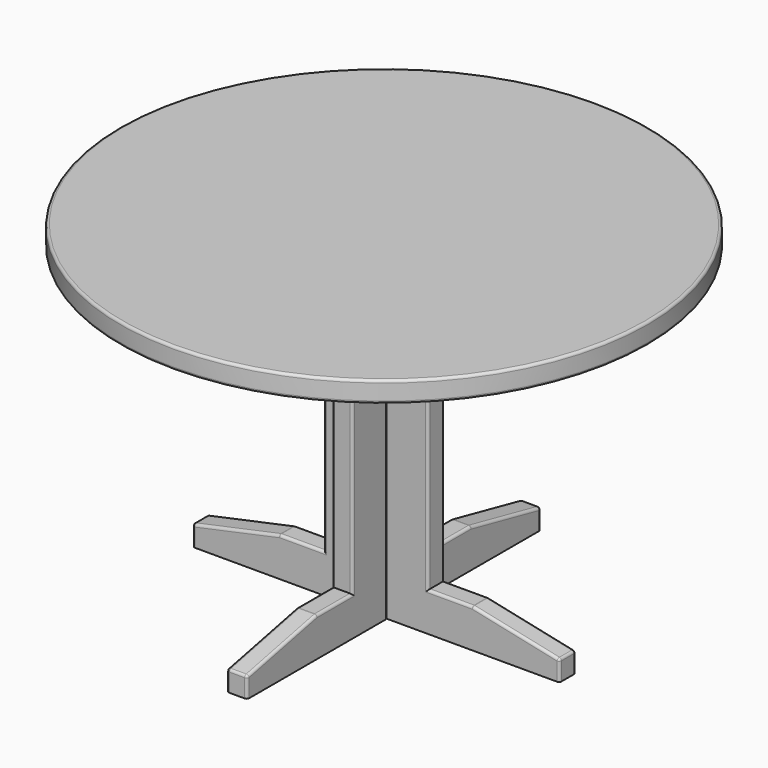
from build123d import *

# Parameters (mm, degrees)
F0_R     = 520.7
F0_W     = 41.275
F0_H     = 256.3125
F0_W_2   = 256.3125
F0_H_2   = 41.275
F0_H_3   = 85
F0_W_3   = 85
F1_DEPTH = 41.275
F2_W     = 82.5
F2_H     = 473.8182766121
F3_DEPTH = 20
F2_H_2   = 474.3196274297
F4_W     = 82.5
F4_H     = 474.3196274297
F5_DEPTH = 20
F4_H_2   = 473.6138966055
F6_R     = 5.08
F6_2_R   = 5.08
F6_3_R   = 5.08
F6_4_R   = 5.08
F6_5_R   = 5.08


# Not quite as in the source:
# - a feature names something its author has since deleted; it is built from what else it names


with BuildPart() as f1:
    # F0 (on Top) → F1 (new body)
    with BuildSketch(Plane.XY):
        Circle(F0_R)
        Polygon((-20.6375, 361.95), (20.6375, 361.95), (20.6375, 105.6375), (20.6375, 20.6375), (105.6375, 20.6375), (361.95, 20.6375), (361.95, -20.6375), (105.6375, -20.6375), (20.6375, -20.6375), (20.6375, -105.6375), (20.6375, -361.95), (-20.6375, -361.95), (-20.6375, -105.6375), (-20.6375, -20.6375), (-105.6375, -20.6375), (-361.95, -20.6375), (-361.95, 20.6375), (-105.6375, 20.6375), (-20.6375, 20.6375), (-20.6375, 105.6375), align=None, mode=Mode.SUBTRACT)
        with Locations((0, 233.79375)):
            Rectangle(F0_W, F0_H)
        with Locations((-233.79375, 0)):
            Rectangle(F0_W_2, F0_H_2)
        with Locations((0, -233.79375)):
            Rectangle(F0_W, F0_H)
        with Locations((233.79375, 0)):
            Rectangle(F0_W_2, F0_H_2)
        Rectangle(F0_W, F0_H_2)
        with Locations((0, 63.1375)):
            Rectangle(F0_W, F0_H_3)
        with Locations((63.1375, 0)):
            Rectangle(F0_W_3, F0_H_2)
        with Locations((0, -63.1375)):
            Rectangle(F0_W, F0_H_3)
        with Locations((-63.1375, 0)):
            Rectangle(F0_W_3, F0_H_2)
    extrude(amount=F1_DEPTH)

    # F6
    f6_edges = [f1.edges().sort_by_distance(p)[0] for p in [
        (-520.7, 0, 41.275),
        (-520.7, 0, 0),
    ]]
    fillet(f6_edges, radius=F6_R)


with BuildPart() as f3:
    # F2 (on Front) → F3 (new body, symmetric)
    with BuildSketch(Plane.XZ):
        Polygon((-361.8104448189, -628.6917154359), (-190.2660957707, -628.7684989539), (-190.2660957707, -551.8782992659), (-361.8104448189, -588.6917154359), align=None)
        Polygon((-190.2660957707, -628.7684989539), (-20.2660957707, -628.8445912188), (-20.2660957707, -551.8782992659), (-102.7660957707, -551.8782992659), (-190.2660957707, -551.8782992659), align=None)
        Polygon((-102.7660957707, -78.0600226537), (-20.2660957707, -78.0600226537), (-20.2660957707, 0), (-190.2660957707, 0), (-190.2660957707, -78.0600226537), align=None)
        Polygon((-362.0399236679, -40), (-190.2660957707, -78.0600226537), (-190.2660957707, 0), (-362.0399236679, 0), align=None)
        with Locations((-61.5160957707, -314.9691609598)):
            Rectangle(F2_W, F2_H)
    extrude(amount=F3_DEPTH, both=True)

    # F6#4
    f6_4_edges = [f3.edges().sort_by_distance(p)[0] for p in [
        (-276.03827, 20, -570.285007),
        (-146.516096, 20, -551.878299),
        (-102.766096, 20, -314.969161),
        (-146.516096, 20, -78.060023),
        (-276.15301, 20, -59.030011),
        (-276.15301, -20, -59.030011),
        (-146.516096, -20, -78.060023),
        (-362.039924, 20, -20),
        (-361.810445, 20, -608.691715),
        (-361.810445, -20, -608.691715),
        (-361.810445, 0, -588.691715),
        (-362.039924, 0, -40),
        (-362.039924, -20, -20),
        (-276.03827, -20, -570.285007),
        (-146.516096, -20, -551.878299),
        (-190.266096, 0, -551.878299),
        (-102.766096, -20, -314.969161),
    ]]
    fillet(f6_4_edges, radius=F6_4_R)


with BuildPart() as f3b:
    # F2 (on Front) → F3, piece 2 (new body, symmetric)
    with BuildSketch(Plane.XZ):
        Polygon((103.0506108094, -552.45), (20.5506108094, -552.45), (20.5506108094, -628.8628608403), (190.5506108094, -628.9389531052), (190.5506108094, -552.45), align=None)
        Polygon((362.153455615, -589.0157628059), (190.5506108094, -552.45), (190.5506108094, -628.9389531052), (362.153455615, -629.0157628059), align=None)
        Polygon((364.0458583832, 0), (190.5506108094, 0), (190.5506108094, -78.1303725703), (364.0458583832, -40), align=None)
        Polygon((190.5506108094, 0), (20.5506108094, 0), (20.5506108094, -78.1303725703), (103.0506108094, -78.1303725703), (190.5506108094, -78.1303725703), align=None)
        with Locations((61.8006108094, -315.2901862851)):
            Rectangle(F2_W, F2_H_2)
    extrude(amount=F3_DEPTH, both=True)

    # F6#2
    f6_2_edges = [f3b.edges().sort_by_distance(p)[0] for p in [
        (277.298235, -20, -59.065186),
        (146.800611, -20, -78.130373),
        (364.045858, -20, -20),
        (364.045858, 20, -20),
        (364.045858, 0, -40),
        (277.298235, 20, -59.065186),
        (146.800611, 20, -78.130373),
        (103.050611, 20, -315.290186),
        (103.050611, -20, -315.290186),
        (146.800611, -20, -552.45),
        (276.352033, -20, -570.732881),
        (362.153456, 20, -609.015763),
        (362.153456, -20, -609.015763),
        (362.153456, 0, -589.015763),
        (276.352033, 20, -570.732881),
        (146.800611, 20, -552.45),
        (190.550611, 0, -552.45),
    ]]
    fillet(f6_2_edges, radius=F6_2_R)


with BuildPart() as f5:
    # F4 (on Right) → F5 (new body, symmetric)
    with BuildSketch(Plane.YZ):
        Polygon((102.507681396, -553.9537763821), (20.007681396, -553.9537763821), (20.007681396, -630.3666372223), (190.007681396, -630.4427294873), (190.007681396, -553.9537763821), align=None)
        Polygon((361.6105262016, -590.519539188), (190.007681396, -553.9537763821), (190.007681396, -630.4427294873), (361.6105262016, -630.519539188), align=None)
        Polygon((190.007681396, -1.5037763821), (20.007681396, -1.5037763821), (20.007681396, -79.6341489524), (102.507681396, -79.6341489524), (190.007681396, -79.6341489524), align=None)
        Polygon((363.5029289697, -1.5037763821), (190.007681396, -1.5037763821), (190.007681396, -79.6341489524), (363.5029289697, -41.5037763821), align=None)
        with Locations((61.257681396, -316.7939626672)):
            Rectangle(F4_W, F4_H)
    extrude(amount=F5_DEPTH, both=True)

    # F6#3
    f6_3_edges = [f5.edges().sort_by_distance(p)[0] for p in [
        (20, 146.257681, -79.634149),
        (20, 102.507681, -316.793963),
        (20, 276.755305, -60.568963),
        (20, 363.502929, -21.503776),
        (-20, 363.502929, -21.503776),
        (-20, 276.755305, -60.568963),
        (-20, 146.257681, -79.634149),
        (-20, 102.507681, -316.793963),
        (20, 146.257681, -553.953776),
        (20, 275.809104, -572.236658),
        (-20, 361.610526, -610.519539),
        (0, 361.610526, -590.519539),
        (20, 361.610526, -610.519539),
        (-20, 275.809104, -572.236658),
        (-20, 146.257681, -553.953776),
        (0, 190.007681, -553.953776),
        (0, 363.502929, -41.503776),
    ]]
    fillet(f6_3_edges, radius=F6_3_R)


with BuildPart() as f5b:
    # F4 (on Right) → F5, piece 2 (new body, symmetric)
    with BuildSketch(Plane.YZ):
        Polygon((-190.3404469946, -630.2724850723), (-20.3404469946, -630.3485773372), (-20.3404469946, -553.2815187716), (-102.8404469946, -553.2815187716), (-190.3404469946, -553.2815187716), align=None)
        Polygon((-362.3533742323, -630.195491818), (-190.3404469946, -630.2724850723), (-190.3404469946, -553.2815187716), (-362.3533742323, -590.195491818), align=None)
        Polygon((-102.8404469946, -79.6676221661), (-20.3404469946, -79.6676221661), (-20.3404469946, -1.5037763821), (-190.3404469946, -1.5037763821), (-190.3404469946, -79.6676221661), align=None)
        Polygon((-362.5828530813, -41.5037763821), (-190.3404469946, -79.6676221661), (-190.3404469946, -1.5037763821), (-362.5828530813, -1.5037763821), align=None)
        with Locations((-61.5904469946, -316.4745704688)):
            Rectangle(F4_W, F4_H_2)
    extrude(amount=F5_DEPTH, both=True)

    # F6#5
    f6_5_edges = [f5b.edges().sort_by_distance(p)[0] for p in [
        (20, -102.840447, -316.47457),
        (-20, -102.840447, -316.47457),
        (20, -146.590447, -79.667622),
        (-20, -146.590447, -79.667622),
        (0, -190.340447, -79.667622),
        (20, -276.46165, -60.585699),
        (-20, -276.46165, -60.585699),
        (20, -276.346911, -571.738505),
        (20, -146.590447, -553.281519),
        (20, -362.353374, -610.195492),
        (0, -362.353374, -590.195492),
        (-20, -362.353374, -610.195492),
        (-20, -146.590447, -553.281519),
        (-20, -276.346911, -571.738505),
        (0, -190.340447, -553.281519),
        (0, -362.582853, -41.503776),
        (20, -362.582853, -21.503776),
        (-20, -362.582853, -21.503776),
    ]]
    fillet(f6_5_edges, radius=F6_5_R)


solid = Compound([f1.part, f3.part, f3b.part, f5.part, f5b.part])
